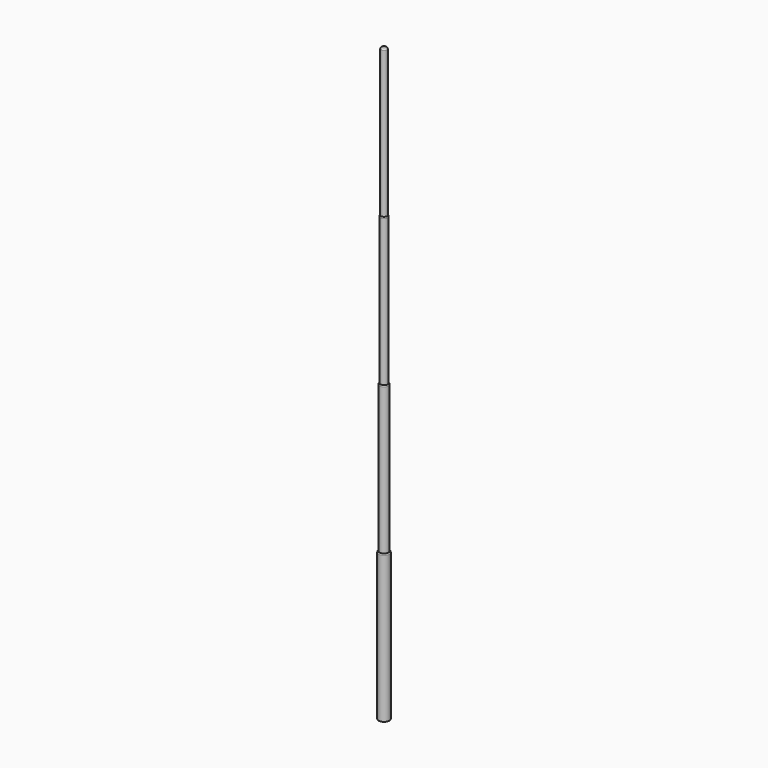
from build123d import *

# Parameters (mm, degrees)
F0_R     = 7.1577178439
F0_R_2   = 6
F0_R_3   = 5
F0_R_4   = 4
F1_DEPTH = 200
F2_DEPTH = 400
F3_DEPTH = 600
F4_DEPTH = 800


# Not quite as in the source:
# - a fillet or chamfer that OpenCascade refuses, or shapes differently, is made with other operations: its cross-section is extruded or revolved along the edge and cut away or added


with BuildPart() as f1:
    # F0 (on Top) → F1 (new body)
    with BuildSketch(Plane.XY):
        with Locations((231.38127774, 15.8246317059)):
            Circle(F0_R)
        with Locations((231.38127774, 15.8246317059)):
            Circle(F0_R_2, mode=Mode.SUBTRACT)
        with Locations((231.38127774, 15.8246317059)):
            Circle(F0_R_2)
        with Locations((231.38127774, 15.8246317059)):
            Circle(F0_R_3, mode=Mode.SUBTRACT)
        with Locations((231.38127774, 15.8246317059)):
            Circle(F0_R_3)
        with Locations((231.38127774, 15.8246317059)):
            Circle(F0_R_4, mode=Mode.SUBTRACT)
        with Locations((231.38127774, 15.8246317059)):
            Circle(F0_R_4)
    extrude(amount=F1_DEPTH)

    # F0 (on Top) → F2 (join)
    with BuildSketch(Plane.XY):
        with Locations((231.38127774, 15.8246317059)):
            Circle(F0_R_2)
        with Locations((231.38127774, 15.8246317059)):
            Circle(F0_R_3, mode=Mode.SUBTRACT)
        with Locations((231.38127774, 15.8246317059)):
            Circle(F0_R_3)
        with Locations((231.38127774, 15.8246317059)):
            Circle(F0_R_4, mode=Mode.SUBTRACT)
        with Locations((231.38127774, 15.8246317059)):
            Circle(F0_R_4)
    extrude(amount=F2_DEPTH)

    # F0 (on Top) → F3 (join)
    with BuildSketch(Plane.XY):
        with Locations((231.38127774, 15.8246317059)):
            Circle(F0_R_3)
        with Locations((231.38127774, 15.8246317059)):
            Circle(F0_R_4, mode=Mode.SUBTRACT)
        with Locations((231.38127774, 15.8246317059)):
            Circle(F0_R_4)
    extrude(amount=F3_DEPTH)

    # F0 (on Top) → F4 (join)
    with BuildSketch(Plane.XY):
        with Locations((231.38127774, 15.8246317059)):
            Circle(F0_R_4)
    extrude(amount=F4_DEPTH)

    # F5: fillet of radius 2 on 4 edges, made by hand

    # F5_s1 → F5_t2 (revolve, cut)
    with BuildSketch(Plane.XZ.offset(-15.8246317059)):
        with BuildLine():
            ThreePointArc((238.5393955839, 198.1853934994), (238.2252538415, 199.261841349), (237.3814463082, 200.0003627462))
            Line((237.3814463082, 200.0003627462), (237.4657879491, 200.1818596708))
            ThreePointArc((237.4657879491, 200.1818596708), (237.9602209461, 200.2001365685), (238.5389955839, 200.2001365685))
            Line((238.5389955839, 200.2001365685), (238.7391321525, 200))
            ThreePointArc((238.7391321525, 200), (238.7391321525, 199.0926967497), (238.7395321525, 198.1853934994))
            Line((238.7395321525, 198.1853934994), (238.5393955839, 198.1853934994))
        make_face()
    revolve(axis=Axis((231.38127774, 15.8246317059, 200), (0, 0, 1)), mode=Mode.SUBTRACT)

    # F5_s3 → F5_t4 (revolve, cut)
    with BuildSketch(Plane.XZ.offset(-15.8246317059)):
        with BuildLine():
            ThreePointArc((237.38167774, 398.2673917434), (237.1136849874, 399.2678330874), (236.3814778365, 400.0003463544))
            Line((236.3814778365, 400.0003463544), (236.4815944147, 400.1736418155))
            ThreePointArc((236.4815944147, 400.1736418155), (236.8813777883, 400.2001365685), (237.38127774, 400.2001365685))
            Line((237.38127774, 400.2001365685), (237.5814143085, 400))
            ThreePointArc((237.5814143085, 400), (237.5814143085, 399.1336958717), (237.5818143085, 398.2673917434))
            Line((237.5818143085, 398.2673917434), (237.38167774, 398.2673917434))
        make_face()
    revolve(axis=Axis((231.38127774, 15.8246317059, 400), (0, 0, 1)), mode=Mode.SUBTRACT)

    # F5_s5 → F5_t6 (revolve, cut)
    with BuildSketch(Plane.XZ.offset(-15.8246317059)):
        with BuildLine():
            ThreePointArc((236.38167774, 598.2673917434), (236.1136849874, 599.2678330874), (235.3814778365, 600.0003463544))
            Line((235.3814778365, 600.0003463544), (235.4815944147, 600.1736418155))
            ThreePointArc((235.4815944147, 600.1736418155), (235.8813777883, 600.2001365685), (236.38127774, 600.2001365685))
            Line((236.38127774, 600.2001365685), (236.5814143085, 600))
            ThreePointArc((236.5814143085, 600), (236.5814143085, 599.1336958717), (236.5818143085, 598.2673917434))
            Line((236.5818143085, 598.2673917434), (236.38167774, 598.2673917434))
        make_face()
    revolve(axis=Axis((231.38127774, 15.8246317059, 600), (0, 0, 1)), mode=Mode.SUBTRACT)

    # F5_s7 → F5_t8 (revolve, cut)
    with BuildSketch(Plane.XZ.offset(-15.8246317059)):
        with BuildLine():
            ThreePointArc((235.38167774, 797.9990343146), (234.7954913024, 799.4142135624), (233.3803120546, 800.0004))
            Line((233.3803120546, 800.0004), (233.3803120546, 800.2005365685))
            ThreePointArc((233.3803120546, 800.2005365685), (234.3807948973, 800.2001365685), (235.38127774, 800.2001365685))
            Line((235.38127774, 800.2001365685), (235.5814143085, 800))
            ThreePointArc((235.5814143085, 800), (235.5814143085, 798.9995171573), (235.5818143085, 797.9990343146))
            Line((235.5818143085, 797.9990343146), (235.38167774, 797.9990343146))
        make_face()
    revolve(axis=Axis((231.38127774, 15.8246317059, 800), (0, 0, 1)), mode=Mode.SUBTRACT)


solid = f1.part
